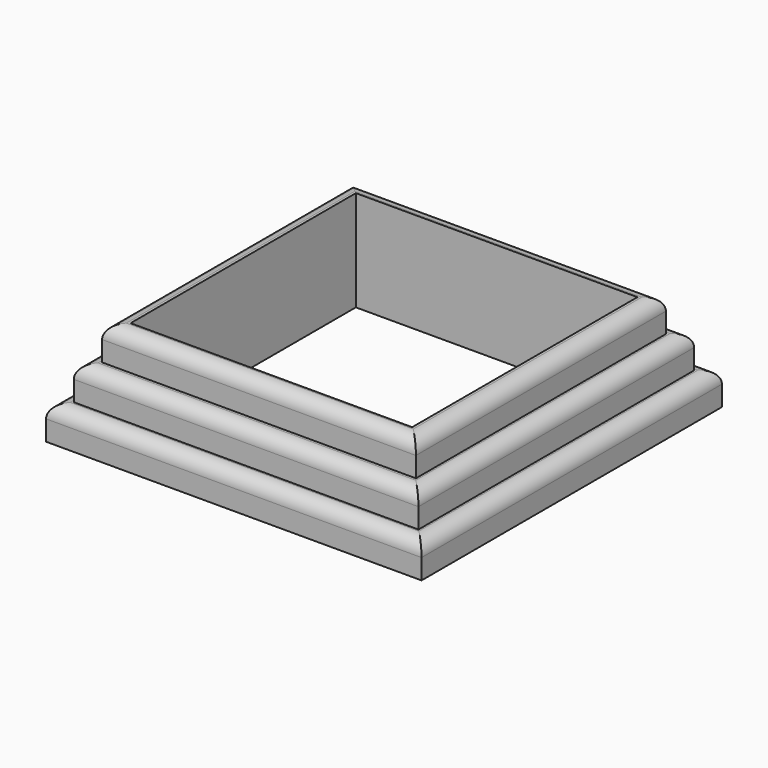
from build123d import *

# Parameters (mm, degrees)
F0_W     = 142.24
F0_H     = 142.24
F1_DEPTH = 12.7
F2_W     = 106.68
F2_H     = 106.68
F3_DEPTH = 12.701
F4_W     = 130.556
F4_H     = 130.556
F4_W_2   = 106.68
F4_H_2   = 106.68
F5_DEPTH = 12.7
F6_W     = 118.872
F6_H     = 118.364
F6_W_2   = 106.68
F6_H_2   = 106.68
F7_DEPTH = 12.7
F8_R     = 5.08


with BuildPart() as f1:
    # F0 (on Top) → F1 (new body)
    with BuildSketch(Plane.XY):
        Rectangle(F0_W, F0_H)
    extrude(amount=F1_DEPTH)

    # F2 (on face) → F3 (cut, through all)
    with BuildSketch(Plane.XY.offset(12.7)):
        Rectangle(F2_W, F2_H)
    extrude(amount=-F3_DEPTH, mode=Mode.SUBTRACT)

    # F4 (on face) → F5 (join)
    with BuildSketch(Plane.XY.offset(12.7)):
        Rectangle(F4_W, F4_H)
        Rectangle(F4_W_2, F4_H_2, mode=Mode.SUBTRACT)
    extrude(amount=F5_DEPTH)

    # F6 (on face) → F7 (join)
    with BuildSketch(Plane.XY.offset(25.4)):
        Rectangle(F6_W, F6_H)
        Rectangle(F6_W_2, F6_H_2, mode=Mode.SUBTRACT)
    extrude(amount=F7_DEPTH)

    # F8
    f8_edges = [f1.edges().sort_by_distance(p)[0] for p in [
        (0, -59.182, 38.1),
        (-59.436, 0, 38.1),
        (0, -65.278, 25.4),
        (0, -71.12, 12.7),
        (-71.12, 0, 12.7),
        (-65.278, 0, 25.4),
        (0, 71.12, 12.7),
        (0, 65.278, 25.4),
        (0, 59.182, 38.1),
        (59.436, 0, 38.1),
        (65.278, 0, 25.4),
        (71.12, 0, 12.7),
    ]]
    fillet(f8_edges, radius=F8_R)


solid = f1.part
